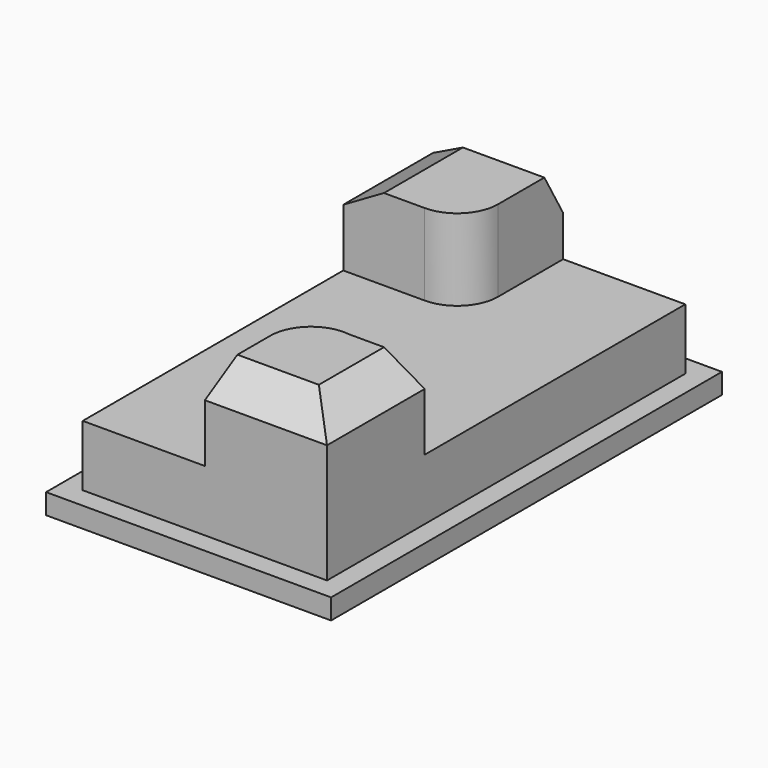
from build123d import *

# Parameters (mm, degrees)
F0_W        = 88.9
F0_H        = 152.4
F1_DEPTH    = 6.35
F2_DEPTH    = 25.4
F3_DEPTH    = 50.8
F4_C1_SIZE2 = 12.7
F4_C1_SIZE  = 7.3323484187
F4_C2_SIZE2 = 12.7
F4_C2_SIZE  = 7.3323484187
F4_C3_SIZE2 = 7.3323484187
F4_C3_SIZE  = 12.7
F4_C4_SIZE2 = 12.7
F4_C4_SIZE  = 7.3323484187


with BuildPart() as f1:
    # F0 (on Top) → F1 (new body)
    with BuildSketch(Plane.XY):
        with Locations((-31.1787627001, 11.3253805135)):
            Rectangle(F0_W, F0_H)
        Polygon((-69.2787627001, 43.0753805135), (-69.2787627001, 81.1753805135), (-31.1787627001, 81.1753805135), (6.9212372999, 81.1753805135), (6.9212372999, -20.4246194865), (6.9212372999, -58.5246194865), (-31.1787627001, -58.5246194865), (-69.2787627001, -58.5246194865), align=None, mode=Mode.SUBTRACT)
    extrude(amount=F1_DEPTH)

    # F0 (on Top) → F2 (join)
    with BuildSketch(Plane.XY):
        with BuildLine():
            Line((6.9212372999, 81.1753805135), (-31.1787627001, 81.1753805135))
            Line((-31.1787627001, 81.1753805135), (-31.1787627001, 55.7753805135))
            ThreePointArc((-31.1787627001, 55.7753805135), (-34.898506579, 46.7951243925), (-43.8787627001, 43.0753805135))
            Line((-43.8787627001, 43.0753805135), (-69.2787627001, 43.0753805135))
            Line((-69.2787627001, 43.0753805135), (-69.2787627001, -58.5246194865))
            Line((-69.2787627001, -58.5246194865), (-31.1787627001, -58.5246194865))
            Line((-31.1787627001, -58.5246194865), (-31.1787627001, -33.0056861837))
            ThreePointArc((-31.1787627001, -33.0056861837), (-26.8234670857, -23.4319769383), (-16.7447613275, -20.4246194865))
            Line((-16.7447613275, -20.4246194865), (6.9212372999, -20.4246194865))
            Line((6.9212372999, -20.4246194865), (6.9212372999, 81.1753805135))
        make_face()
    extrude(amount=F2_DEPTH)

    # F0 (on Top) → F3 (join)
    with BuildSketch(Plane.XY):
        with BuildLine():
            Line((-31.1787627001, 81.1753805135), (-69.2787627001, 81.1753805135))
            Line((-69.2787627001, 81.1753805135), (-69.2787627001, 43.0753805135))
            Line((-69.2787627001, 43.0753805135), (-43.8787627001, 43.0753805135))
            ThreePointArc((-43.8787627001, 43.0753805135), (-34.898506579, 46.7951243925), (-31.1787627001, 55.7753805135))
            Line((-31.1787627001, 55.7753805135), (-31.1787627001, 81.1753805135))
        make_face()
        with BuildLine():
            Line((6.9212372999, -58.5246194865), (6.9212372999, -20.4246194865))
            Line((6.9212372999, -20.4246194865), (-16.7447613275, -20.4246194865))
            ThreePointArc((-16.7447613275, -20.4246194865), (-26.8234670857, -23.4319769383), (-31.1787627001, -33.0056861837))
            Line((-31.1787627001, -33.0056861837), (-31.1787627001, -58.5246194865))
            Line((-31.1787627001, -58.5246194865), (6.9212372999, -58.5246194865))
        make_face()
    extrude(amount=F3_DEPTH)

    # F4: chamfer of 12.7 x 7.3323484187 on 4 edges, made by hand

    # F4_c1
    f4_c1_edges = [f1.edges().sort_by_distance(p)[0] for p in [
        (-12.1287627001, -58.5246194865, 50.8),
    ]]
    f4_c1_side = f1.faces().sort_by_distance((-12.1287627001, -58.5246194865, 50.6533530316))[0]
    chamfer(f4_c1_edges, length=F4_C1_SIZE, length2=F4_C1_SIZE2, reference=f4_c1_side)

    # F4_c2
    f4_c2_edges = [f1.edges().sort_by_distance(p)[0] for p in [
        (6.9212372999, -33.1246194865, 50.8),
    ]]
    f4_c2_side = f1.faces().sort_by_distance((6.9212372999, -33.1246194865, 50.6533530316))[0]
    chamfer(f4_c2_edges, length=F4_C2_SIZE, length2=F4_C2_SIZE2, reference=f4_c2_side)

    # F4_c3
    f4_c3_edges = [f1.edges().sort_by_distance(p)[0] for p in [
        (-50.2287627001, 81.1753805135, 50.8),
    ]]
    f4_c3_side = f1.faces().sort_by_distance((-50.2287627001, 81.1753805135, 50.6533530316))[0]
    chamfer(f4_c3_edges, length=F4_C3_SIZE, length2=F4_C3_SIZE2, reference=f4_c3_side)

    # F4_c4
    f4_c4_edges = [f1.edges().sort_by_distance(p)[0] for p in [
        (-69.2787627001, 58.4592063042, 50.8),
    ]]
    f4_c4_side = f1.faces().sort_by_distance((-69.2787627001, 58.4592063042, 50.6533530316))[0]
    chamfer(f4_c4_edges, length=F4_C4_SIZE, length2=F4_C4_SIZE2, reference=f4_c4_side)


solid = f1.part
